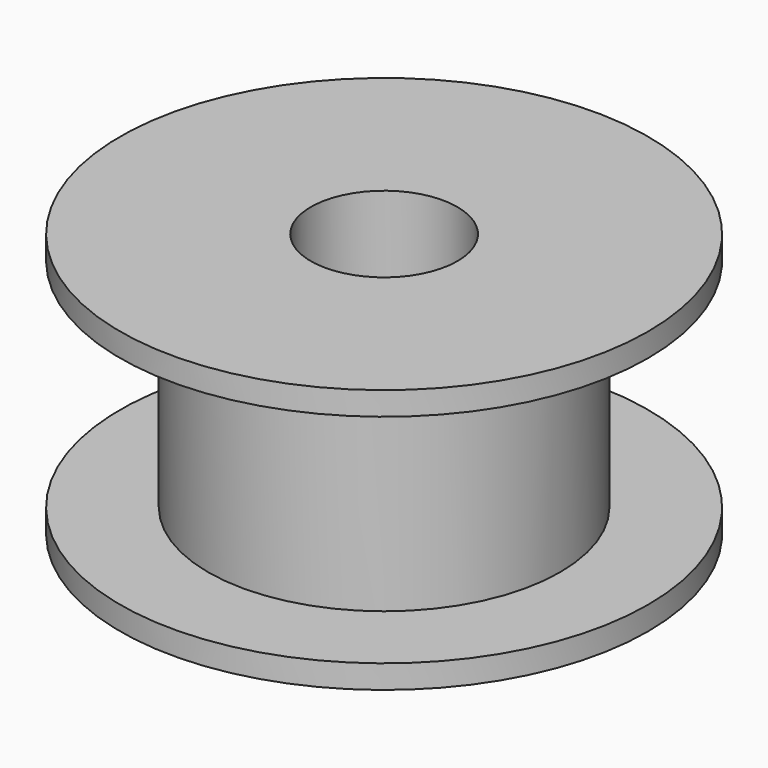
from build123d import *

# Parameters (mm, degrees)
F0_R     = 6
F1_DEPTH = 7.4
F2_R     = 9
F3_DEPTH = 0.8
F4_R     = 9
F5_DEPTH = 0.8
F6_R     = 2.5
F7_DEPTH = 9.001


# Not quite as in the source:
# - ends of sketch curves that miss each other by under 0.0002 mm in the source are joined


with BuildPart() as f1:
    # F0 (on Top) → F1 (new body)
    with BuildSketch(Plane.XY):
        Circle(F0_R)
        with BuildLine():
            ThreePointArc((0.3806045388, -5.7658808945), (0.3821052842, -5.7646171302), (0.3836035472, -5.7633504238))
            ThreePointArc((0.3836035472, -5.7633504238), (0, -5.25), (-0.3836035472, -5.7633504238))
            ThreePointArc((-0.3836035472, -5.7633504238), (-0.3821052842, -5.7646171302), (-0.3806045388, -5.7658808945))
            ThreePointArc((-0.3806045388, -5.7658808945), (-0.3463448965, -5.8591249109), (-0.4093829562, -5.9358997292))
            ThreePointArc((-0.4093829562, -5.9358997292), (-0.4525361238, -5.9421469593), (-0.4942455569, -5.9294368476))
            ThreePointArc((-0.4942455569, -5.9294368476), (-0.9311233557, -5.8766920369), (-1.3629081057, -5.7918029572))
            ThreePointArc((-1.3629081057, -5.7918029572), (-1.4044855806, -5.7906197903), (-1.441985055, -5.7726232426))
            ThreePointArc((-1.441985055, -5.7726232426), (-1.4799897199, -5.6798690996), (-1.4184467175, -5.6007480248))
            ThreePointArc((-1.4184467175, -5.6007480248), (-1.4166288992, -5.6000098693), (-1.4148125327, -5.5992681488))
            ThreePointArc((-1.4148125327, -5.5992681488), (-1.6210071809, -4.9925028678), (-2.1444698391, -5.3621881184))
            ThreePointArc((-2.1444698391, -5.3621881184), (-2.1434363401, -5.3638558164), (-2.1423995711, -5.3655214836))
            ThreePointArc((-2.1423995711, -5.3655214836), (-2.1392066719, -5.4658737363), (-2.2247634424, -5.5184171304))
            ThreePointArc((-2.2247634424, -5.5184171304), (-2.2652635999, -5.5109390447), (-2.2993151455, -5.4877727597))
            ThreePointArc((-2.2993151455, -5.4877727597), (-2.7009268548, -5.3016501323), (-3.0875904018, -5.0861857527))
            ThreePointArc((-3.0875904018, -5.0861857527), (-3.1238007071, -5.0726605298), (-3.1521764439, -5.0464129504))
            ThreePointArc((-3.1521764439, -5.0464129504), (-3.1620439351, -4.945353315), (-3.078417275, -4.8877599211))
            ThreePointArc((-3.078417275, -4.8877599211), (-3.0764603245, -4.8876196303), (-3.0745036529, -4.8874755002))
            ThreePointArc((-3.0745036529, -4.8874755002), (-3.0831056333, -4.2466897755), (-3.6951872305, -4.4365224847))
            ThreePointArc((-3.6951872305, -4.4365224847), (-3.6947196616, -4.4384279285), (-3.6942483551, -4.4403324513))
            ThreePointArc((-3.6942483551, -4.4403324513), (-3.7234373447, -4.5379012507), (-3.8230076712, -4.5592885789))
            ThreePointArc((-3.8230076712, -4.5592885789), (-3.8560268582, -4.5406730269), (-3.8797455624, -4.5111056706))
            ThreePointArc((-3.8797455624, -4.5111056706), (-4.2068112489, -4.2077593938), (-4.5102312248, -3.8807620771))
            ThreePointArc((-4.5102312248, -3.8807620771), (-4.5371123267, -3.8585413389), (-4.5547275545, -3.8284405316))
            ThreePointArc((-4.5547275545, -3.8284405316), (-4.535446501, -3.7270635192), (-4.4368176497, -3.6967088266))
            ThreePointArc((-4.4368176497, -3.6967088266), (-4.4349131269, -3.6971801331), (-4.433007683, -3.697647702))
            ThreePointArc((-4.433007683, -3.697647702), (-4.2431749738, -3.0855661048), (-4.8839606986, -3.0769641244))
            ThreePointArc((-4.8839606986, -3.0769641244), (-4.8841048286, -3.0789207959), (-4.8842451195, -3.0808777465))
            ThreePointArc((-4.8842451195, -3.0808777465), (-4.9440169669, -3.1654857116), (-5.0466911586, -3.1517310085))
            ThreePointArc((-5.0466911586, -3.1517310085), (-5.069110444, -3.1263184325), (-5.0817550004, -3.0948773992))
            ThreePointArc((-5.0817550004, -3.0948773992), (-5.3012375926, -2.7017364763), (-5.4903626511, -2.2931240611))
            ThreePointArc((-5.4903626511, -2.2931240611), (-5.5060730233, -2.2671022941), (-5.5132397924, -2.2375627347))
            ThreePointArc((-5.5132397924, -2.2375627347), (-5.4658096238, -2.1437373386), (-5.3606781484, -2.144183121))
            ThreePointArc((-5.3606781484, -2.144183121), (-5.3590124813, -2.14521989), (-5.3573447832, -2.146253389))
            ThreePointArc((-5.3573447832, -2.146253389), (-4.9876595327, -1.6227907307), (-5.5944248136, -1.4165960825))
            ThreePointArc((-5.5944248136, -1.4165960825), (-5.5951665342, -1.4184124491), (-5.5959046897, -1.4202302674))
            ThreePointArc((-5.5959046897, -1.4202302674), (-5.6812065984, -1.4824247971), (-5.7747415985, -1.4334781025))
            ThreePointArc((-5.7747415985, -1.4334781025), (-5.7857648681, -1.4063168524), (-5.7884387811, -1.3771261661))
            ThreePointArc((-5.7884387811, -1.3771261661), (-5.8767455172, -0.9307857571), (-5.9306876982, -0.4790025331))
            ThreePointArc((-5.9306876982, -0.4790025331), (-5.8853739929, -0.3594639118), (-5.7595648686, -0.3821548374))
            ThreePointArc((-5.7595648686, -0.3821548374), (-5.7583011043, -0.3836555828), (-5.7570343979, -0.3851538458))
            ThreePointArc((-5.7570343979, -0.3851538458), (-5.2436839741, -0.0015502986), (-5.7570343979, 0.3820532486))
            ThreePointArc((-5.7570343979, 0.3820532486), (-5.7583011043, 0.3805549856), (-5.7595648686, 0.3790542403))
            ThreePointArc((-5.7595648686, 0.3790542403), (-5.8622942172, 0.3468784197), (-5.9346909264, 0.426548483))
            ThreePointArc((-5.9346909264, 0.426548483), (-5.9358323151, 0.4509676612), (-5.9310148859, 0.4749341254))
            ThreePointArc((-5.9310148859, 0.4749341254), (-5.8765991635, 0.9317093277), (-5.7870583583, 1.3829156003))
            ThreePointArc((-5.7870583583, 1.3829156003), (-5.7843038364, 1.4029349854), (-5.7775807433, 1.4219918266))
            ThreePointArc((-5.7775807433, 1.4219918266), (-5.6843404021, 1.4793255219), (-5.594431999, 1.416896419))
            ThreePointArc((-5.594431999, 1.416896419), (-5.5936938435, 1.4150786007), (-5.5929521229, 1.4132622341))
            ThreePointArc((-5.5929521229, 1.4132622341), (-4.986186842, 1.6194568823), (-5.3558720925, 2.1429195405))
            ThreePointArc((-5.3558720925, 2.1429195405), (-5.3575397905, 2.1418860415), (-5.3592054577, 2.1408492726))
            ThreePointArc((-5.3592054577, 2.1408492726), (-5.4688284086, 2.1433207754), (-5.5102834557, 2.2448332315))
            ThreePointArc((-5.5102834557, 2.2448332315), (-5.5046167329, 2.2637285902), (-5.4953509969, 2.2811438842))
            ThreePointArc((-5.4953509969, 2.2811438842), (-5.3005253653, 2.7031335247), (-5.0733549953, 3.1086281688))
            ThreePointArc((-5.0733549953, 3.1086281688), (-5.0663266491, 3.1222793914), (-5.0572912917, 3.1346937317))
            ThreePointArc((-5.0572912917, 3.1346937317), (-4.9499559959, 3.164809758), (-4.8814438952, 3.0768669764))
            ThreePointArc((-4.8814438952, 3.0768669764), (-4.8813036044, 3.0749100259), (-4.8811594743, 3.0729533544))
            ThreePointArc((-4.8811594743, 3.0729533544), (-4.2403737496, 3.0815553348), (-4.4302064588, 3.6936369319))
            ThreePointArc((-4.4302064588, 3.6936369319), (-4.4321119026, 3.693169363), (-4.4340164255, 3.6926980566))
            ThreePointArc((-4.4340164255, 3.6926980566), (-4.538656044, 3.7304491107), (-4.5436525599, 3.841577985))
            ThreePointArc((-4.5436525599, 3.841577985), (-4.5343248359, 3.8545144167), (-4.523059132, 3.8658034209))
            ThreePointArc((-4.523059132, 3.8658034209), (-4.2049856642, 4.2095837756), (-3.8608578947, 4.5272813384))
            ThreePointArc((-3.8608578947, 4.5272813384), (-3.852175731, 4.5356041669), (-3.8425571832, 4.5428244841))
            ThreePointArc((-3.8425571832, 4.5428244841), (-3.729720065, 4.5410442426), (-3.6903928007, 4.4352673511))
            ThreePointArc((-3.6903928007, 4.4352673511), (-3.6908641072, 4.4333628283), (-3.6913316761, 4.4314573845))
            ThreePointArc((-3.6913316761, 4.4314573845), (-3.0792500789, 4.2416246753), (-3.0706480985, 4.8824104))
            ThreePointArc((-3.0706480985, 4.8824104), (-3.0726047701, 4.8825545301), (-3.0745617206, 4.8826948209))
            ThreePointArc((-3.0745617206, 4.8826948209), (-3.1626644803, 4.9516976688), (-3.1315994665, 5.0592079204))
            ThreePointArc((-3.1315994665, 5.0592079204), (-3.119936027, 5.0676010486), (-3.1071900735, 5.074235888))
            ThreePointArc((-3.1071900735, 5.074235888), (-2.6977366196, 5.3032741897), (-2.2715103211, 5.4993400387))
            ThreePointArc((-2.2715103211, 5.4993400387), (-2.1503267928, 5.4810489954), (-2.1378670951, 5.3591278498))
            ThreePointArc((-2.1378670951, 5.3591278498), (-2.1389038641, 5.3574621827), (-2.1399373631, 5.3557944847))
            ThreePointArc((-2.1399373631, 5.3557944847), (-1.6164747048, 4.9861092341), (-1.4102800566, 5.592874515))
            ThreePointArc((-1.4102800566, 5.592874515), (-1.4120964232, 5.5936162356), (-1.4139142415, 5.5943543911))
            ThreePointArc((-1.4139142415, 5.5943543911), (-1.4763804938, 5.6864908439), (-1.4149370546, 5.7793125137))
            ThreePointArc((-1.4149370546, 5.7793125137), (-1.3999049739, 5.7842378178), (-1.3842842971, 5.7867311139))
            ThreePointArc((-1.3842842971, 5.7867311139), (-0.9264014664, 5.8774382449), (-0.4628171036, 5.9319727181))
            ThreePointArc((-0.4628171036, 5.9319727181), (-0.4476995944, 5.9342860016), (-0.4324061315, 5.9342670093))
            ThreePointArc((-0.4324061315, 5.9342670093), (-0.3449604214, 5.8651285474), (-0.3758388115, 5.7580145701))
            ThreePointArc((-0.3758388115, 5.7580145701), (-0.3773395569, 5.7567508057), (-0.3788378199, 5.7554840994))
            ThreePointArc((-0.3788378199, 5.7554840994), (0.0047657273, 5.2421336756), (0.3883692745, 5.7554840994))
            ThreePointArc((0.3883692745, 5.7554840994), (0.3868710115, 5.7567508057), (0.3853702662, 5.7580145701))
            ThreePointArc((0.3853702662, 5.7580145701), (0.3538873578, 5.8631766757), (0.4378708106, 5.9338662905))
            ThreePointArc((0.4378708106, 5.9338662905), (0.4573929959, 5.9342736516), (0.4766221718, 5.9308794715))
            ThreePointArc((0.4766221718, 5.9308794715), (0.9358457669, 5.8759418565), (1.3894149145, 5.785501378))
            ThreePointArc((1.3894149145, 5.785501378), (1.4093589983, 5.7827272829), (1.4283429976, 5.7760138748))
            ThreePointArc((1.4283429976, 5.7760138748), (1.4856410056, 5.6827706834), (1.4232124448, 5.5928817004))
            ThreePointArc((1.4232124448, 5.5928817004), (1.4213946265, 5.5921435449), (1.41957826, 5.5914018243))
            ThreePointArc((1.41957826, 5.5914018243), (1.6257729082, 4.9846365434), (2.1492355664, 5.3543217939))
            ThreePointArc((2.1492355664, 5.3543217939), (2.1482020674, 5.355989492), (2.1471652984, 5.3576551591))
            ThreePointArc((2.1471652984, 5.3576551591), (2.1484055829, 5.4654463163), (2.2467992931, 5.5094820933))
            ThreePointArc((2.2467992931, 5.5094820933), (2.2701462131, 5.5030245881), (2.2912554418, 5.4911427318))
            ThreePointArc((2.2912554418, 5.4911427318), (2.7064393495, 5.298838179), (3.1056182667, 5.0751980436))
            ThreePointArc((3.1056182667, 5.0751980436), (3.1286854235, 5.0647208158), (3.1483792489, 5.048782834))
            ThreePointArc((3.1483792489, 5.048782834), (3.169420639, 4.9436317748), (3.0831830023, 4.8798935967))
            ThreePointArc((3.0831830023, 4.8798935967), (3.0812260518, 4.8797533058), (3.0792693802, 4.8796091758))
            ThreePointArc((3.0792693802, 4.8796091758), (3.0878713606, 4.238823451), (3.6999529578, 4.4286561602))
            ThreePointArc((3.6999529578, 4.4286561602), (3.6994853889, 4.4305616041), (3.6990140824, 4.4324661269))
            ThreePointArc((3.6990140824, 4.4324661269), (3.7316088821, 4.5330409603), (3.8362478957, 4.5481537004))
            ThreePointArc((3.8362478957, 4.5481537004), (3.8609061096, 4.53271015), (3.8800750956, 4.5108222369))
            ThreePointArc((3.8800750956, 4.5108222369), (4.2117676312, 4.2027982846), (4.5190837616, 3.8704498389))
            ThreePointArc((4.5190837616, 3.8704498389), (4.5419784366, 3.8505567927), (4.5578563234, 3.8247151182))
            ThreePointArc((4.5578563234, 3.8247151182), (4.5416785998, 3.7208726241), (4.441583377, 3.6888425022))
            ThreePointArc((4.441583377, 3.6888425022), (4.4396788542, 3.6893138086), (4.4377734103, 3.6897813775))
            ThreePointArc((4.4377734103, 3.6897813775), (4.2479407012, 3.0776997804), (4.8887264259, 3.0690978))
            ThreePointArc((4.8887264259, 3.0690978), (4.8888705559, 3.0710544715), (4.8890108468, 3.073011422))
            ThreePointArc((4.8890108468, 3.073011422), (4.9489466875, 3.1576907408), (5.0517351443, 3.1436399335))
            ThreePointArc((5.0517351443, 3.1436399335), (5.0739585149, 3.1183183587), (5.0865115484, 3.0870536549))
            ThreePointArc((5.0865115484, 3.0870536549), (5.3044458004, 2.6954322011), (5.4922842876, 2.2885177089))
            ThreePointArc((5.4922842876, 2.2885177089), (5.5108977286, 2.2590924146), (5.5182939971, 2.2250688442))
            ThreePointArc((5.5182939971, 2.2250688442), (5.4685840303, 2.1346836809), (5.3654438757, 2.1363167965))
            ThreePointArc((5.3654438757, 2.1363167965), (5.3637782086, 2.1373535655), (5.3621105105, 2.1383870645))
            ThreePointArc((5.3621105105, 2.1383870645), (4.99242526, 1.6149244063), (5.5991905409, 1.4087297581))
            ThreePointArc((5.5991905409, 1.4087297581), (5.5999322615, 1.4105461246), (5.600670417, 1.4123639429))
            ThreePointArc((5.600670417, 1.4123639429), (5.6817933965, 1.4741605567), (5.7749452179, 1.4326575759))
            ThreePointArc((5.7749452179, 1.4326575759), (5.7905658496, 1.3983050131), (5.7923433498, 1.3606096128))
            ThreePointArc((5.7923433498, 1.3606096128), (5.8777300273, 0.9245483905), (5.9303365162, 0.4833309479))
            ThreePointArc((5.9303365162, 0.4833309479), (5.9406046173, 0.4461148884), (5.9360098784, 0.407782691))
            ThreePointArc((5.9360098784, 0.407782691), (5.8600341125, 0.3404768743), (5.7643305959, 0.374288513))
            ThreePointArc((5.7643305959, 0.374288513), (5.7630668316, 0.3757892583), (5.7618001253, 0.3772875213))
            ThreePointArc((5.7618001253, 0.3772875213), (5.2484497014, -0.0063160259), (5.7618001253, -0.3899195731))
            ThreePointArc((5.7618001253, -0.3899195731), (5.7630668316, -0.3884213101), (5.7643305959, -0.3869205647))
            ThreePointArc((5.7643305959, -0.3869205647), (5.8589130817, -0.352896847), (5.9352813712, -0.4182523696))
            ThreePointArc((5.9352813712, -0.4182523696), (5.9405882849, -0.4589613406), (5.9290914374, -0.4983720771))
            ThreePointArc((5.9290914374, -0.4983720771), (5.8758462536, -0.9364458362), (5.7902789498, -1.3693683519))
            ThreePointArc((5.7902789498, -1.3693683519), (5.7890432658, -1.4109094735), (5.7710268611, -1.4483607867))
            ThreePointArc((5.7710268611, -1.4483607867), (5.6782814399, -1.4863006219), (5.5991977263, -1.4247627434))
            ThreePointArc((5.5991977263, -1.4247627434), (5.5984595708, -1.4229449251), (5.5977178502, -1.4211285585))
            ThreePointArc((5.5977178502, -1.4211285585), (4.9909525693, -1.6273232067), (5.3606378198, -2.150785865))
            ThreePointArc((5.3606378198, -2.150785865), (5.3623055179, -2.149752366), (5.363971185, -2.148715597))
            ThreePointArc((5.363971185, -2.148715597), (5.4965423161, -2.1730904294), (5.4844051341, -2.3073361968))
            ThreePointArc((5.4844051341, -2.3073361968), (5.2993121671, -2.705511145), (5.0853590441, -3.0889518275))
            ThreePointArc((5.0853590441, -3.0889518275), (5.0710792206, -3.130167057), (5.0406318988, -3.1614126685))
            ThreePointArc((5.0406318988, -3.1614126685), (4.9414861677, -3.167246403), (4.8862096226, -3.0847333009))
            ThreePointArc((4.8862096226, -3.0847333009), (4.8860693317, -3.0827763503), (4.8859252016, -3.0808196788))
            ThreePointArc((4.8859252016, -3.0808196788), (4.2451394769, -3.0894216592), (4.4349721861, -3.7015032564))
            ThreePointArc((4.4349721861, -3.7015032564), (4.43687763, -3.7010356874), (4.4387821528, -3.700564381))
            ThreePointArc((4.4387821528, -3.700564381), (4.5338661391, -3.7271588755), (4.5597701404, -3.8224332913))
            ThreePointArc((4.5597701404, -3.8224332913), (4.2049311669, -4.2096382127), (3.8173294995, -4.5640437653))
            ThreePointArc((3.8173294995, -4.5640437653), (3.7218637964, -4.5383274637), (3.695158528, -4.4431336756))
            ThreePointArc((3.695158528, -4.4431336756), (3.6956298345, -4.4412291528), (3.6960974034, -4.4393237089))
            ThreePointArc((3.6960974034, -4.4393237089), (3.0840158062, -4.2494909997), (3.0754138259, -4.8902767244))
            ThreePointArc((3.0754138259, -4.8902767244), (3.0773704974, -4.8904208545), (3.0793274479, -4.8905611454))
            ThreePointArc((3.0793274479, -4.8905611454), (3.1614118111, -4.944984516), (3.1570355374, -5.0433745266))
            ThreePointArc((3.1570355374, -5.0433745266), (2.6997840023, -5.3022322036), (2.2214782118, -5.5197404427))
            ThreePointArc((2.2214782118, -5.5197404427), (2.1386184867, -5.4657888682), (2.1426328224, -5.3669941743))
            ThreePointArc((2.1426328224, -5.3669941743), (2.1436695914, -5.3653285072), (2.1447030904, -5.3636608091))
            ThreePointArc((2.1447030904, -5.3636608091), (1.6212404321, -4.9939755586), (1.4150457839, -5.6007408395))
            ThreePointArc((1.4150457839, -5.6007408395), (1.4168621505, -5.6014825601), (1.4186799688, -5.6022207156))
            ThreePointArc((1.4186799688, -5.6022207156), (1.4799653708, -5.6795779085), (1.4450020565, -5.7718687664))
            ThreePointArc((1.4450020565, -5.7718687664), (0.9728192286, -5.8699337942), (0.4942455569, -5.9294368476))
            ThreePointArc((0.4942455569, -5.9294368476), (0.4525361238, -5.9421469593), (0.4093829562, -5.9358997292))
            ThreePointArc((0.4093829562, -5.9358997292), (0.3463448965, -5.8591249109), (0.3806045388, -5.7658808945))
        make_face(mode=Mode.SUBTRACT)
        with BuildLine():
            ThreePointArc((-0.3836035472, -5.7633504238), (0, -5.25), (0.3836035472, -5.7633504238))
            ThreePointArc((0.3836035472, -5.7633504238), (0.3821052842, -5.7646171302), (0.3806045388, -5.7658808945))
            ThreePointArc((0.3806045388, -5.7658808945), (0.3463448965, -5.8591249109), (0.4093829562, -5.9358997292))
            ThreePointArc((0.4093829562, -5.9358997292), (0.4518258123, -5.9328200238), (0.4942455569, -5.9294368476))
            ThreePointArc((0.4942455569, -5.9294368476), (0.9728192286, -5.8699337942), (1.4450020565, -5.7718687664))
            ThreePointArc((1.4450020565, -5.7718687664), (1.4799653708, -5.6795779085), (1.4186799688, -5.6022207156))
            ThreePointArc((1.4186799688, -5.6022207156), (1.4168621505, -5.6014825601), (1.4150457839, -5.6007408395))
            ThreePointArc((1.4150457839, -5.6007408395), (1.6212404321, -4.9939755586), (2.1447030904, -5.3636608091))
            ThreePointArc((2.1447030904, -5.3636608091), (2.1436695914, -5.3653285072), (2.1426328224, -5.3669941743))
            ThreePointArc((2.1426328224, -5.3669941743), (2.1386184867, -5.4657888682), (2.2214782118, -5.5197404427))
            ThreePointArc((2.2214782118, -5.5197404427), (2.6997840023, -5.3022322036), (3.1570355374, -5.0433745266))
            ThreePointArc((3.1570355374, -5.0433745266), (3.1614118111, -4.944984516), (3.0793274479, -4.8905611454))
            ThreePointArc((3.0793274479, -4.8905611454), (3.0773704974, -4.8904208545), (3.0754138259, -4.8902767244))
            ThreePointArc((3.0754138259, -4.8902767244), (3.0840158062, -4.2494909997), (3.6960974034, -4.4393237089))
            ThreePointArc((3.6960974034, -4.4393237089), (3.6956298345, -4.4412291528), (3.695158528, -4.4431336756))
            ThreePointArc((3.695158528, -4.4431336756), (3.7218637964, -4.5383274637), (3.8173294995, -4.5640437653))
            ThreePointArc((3.8173294995, -4.5640437653), (4.2049311669, -4.2096382127), (4.5597701404, -3.8224332913))
            ThreePointArc((4.5597701404, -3.8224332913), (4.5338661391, -3.7271588755), (4.4387821528, -3.700564381))
            ThreePointArc((4.4387821528, -3.700564381), (4.43687763, -3.7010356874), (4.4349721861, -3.7015032564))
            ThreePointArc((4.4349721861, -3.7015032564), (4.2451394769, -3.0894216592), (4.8859252016, -3.0808196788))
            ThreePointArc((4.8859252016, -3.0808196788), (4.8860693317, -3.0827763503), (4.8862096226, -3.0847333009))
            ThreePointArc((4.8862096226, -3.0847333009), (4.9414861677, -3.167246403), (5.0406318988, -3.1614126685))
            ThreePointArc((5.0406318988, -3.1614126685), (5.0631251009, -3.125262263), (5.0853590441, -3.0889518275))
            ThreePointArc((5.0853590441, -3.0889518275), (5.2993121671, -2.705511145), (5.4844051341, -2.3073361968))
            ThreePointArc((5.4844051341, -2.3073361968), (5.4965423161, -2.1730904294), (5.363971185, -2.148715597))
            ThreePointArc((5.363971185, -2.148715597), (5.3623055179, -2.149752366), (5.3606378198, -2.150785865))
            ThreePointArc((5.3606378198, -2.150785865), (4.9909525693, -1.6273232067), (5.5977178502, -1.4211285585))
            ThreePointArc((5.5977178502, -1.4211285585), (5.5984595708, -1.4229449251), (5.5991977263, -1.4247627434))
            ThreePointArc((5.5991977263, -1.4247627434), (5.6782814399, -1.4863006219), (5.7710268611, -1.4483607867))
            ThreePointArc((5.7710268611, -1.4483607867), (5.7807878325, -1.4088974538), (5.7902789498, -1.3693683519))
            ThreePointArc((5.7902789498, -1.3693683519), (5.8758462536, -0.9364458362), (5.9290914374, -0.4983720771))
            ThreePointArc((5.9290914374, -0.4983720771), (5.9323216642, -0.4583226733), (5.9352813712, -0.4182523696))
            ThreePointArc((5.9352813712, -0.4182523696), (5.8589130817, -0.352896847), (5.7643305959, -0.3869205647))
            ThreePointArc((5.7643305959, -0.3869205647), (5.7630668316, -0.3884213101), (5.7618001253, -0.3899195731))
            ThreePointArc((5.7618001253, -0.3899195731), (5.2484497014, -0.0063160259), (5.7618001253, 0.3772875213))
            ThreePointArc((5.7618001253, 0.3772875213), (5.7630668316, 0.3757892583), (5.7643305959, 0.374288513))
            ThreePointArc((5.7643305959, 0.374288513), (5.8600341125, 0.3404768743), (5.9360098784, 0.407782691))
            ThreePointArc((5.9360098784, 0.407782691), (5.9332934424, 0.4455658494), (5.9303365162, 0.4833309479))
            ThreePointArc((5.9303365162, 0.4833309479), (5.8777300273, 0.9245483905), (5.7923433498, 1.3606096128))
            ThreePointArc((5.7923433498, 1.3606096128), (5.7837564722, 1.3966606856), (5.7749452179, 1.4326575759))
            ThreePointArc((5.7749452179, 1.4326575759), (5.6817933965, 1.4741605567), (5.600670417, 1.4123639429))
            ThreePointArc((5.600670417, 1.4123639429), (5.5999322615, 1.4105461246), (5.5991905409, 1.4087297581))
            ThreePointArc((5.5991905409, 1.4087297581), (4.99242526, 1.6149244063), (5.3621105105, 2.1383870645))
            ThreePointArc((5.3621105105, 2.1383870645), (5.3637782086, 2.1373535655), (5.3654438757, 2.1363167965))
            ThreePointArc((5.3654438757, 2.1363167965), (5.4685840303, 2.1346836809), (5.5182939971, 2.2250688442))
            ThreePointArc((5.5182939971, 2.2250688442), (5.5053805482, 2.2568307467), (5.4922842876, 2.2885177089))
            ThreePointArc((5.4922842876, 2.2885177089), (5.3044458004, 2.6954322011), (5.0865115484, 3.0870536549))
            ThreePointArc((5.0865115484, 3.0870536549), (5.0692023043, 3.1153953197), (5.0517351443, 3.1436399335))
            ThreePointArc((5.0517351443, 3.1436399335), (4.9489466875, 3.1576907408), (4.8890108468, 3.073011422))
            ThreePointArc((4.8890108468, 3.073011422), (4.8888705559, 3.0710544715), (4.8887264259, 3.0690978))
            ThreePointArc((4.8887264259, 3.0690978), (4.2479407012, 3.0776997804), (4.4377734103, 3.6897813775))
            ThreePointArc((4.4377734103, 3.6897813775), (4.4396788542, 3.6893138086), (4.441583377, 3.6888425022))
            ThreePointArc((4.441583377, 3.6888425022), (4.5416785998, 3.7208726241), (4.5578563234, 3.8247151182))
            ThreePointArc((4.5578563234, 3.8247151182), (4.5385276514, 3.8476313177), (4.5190837616, 3.8704498389))
            ThreePointArc((4.5190837616, 3.8704498389), (4.2117676312, 4.2027982846), (3.8800750956, 4.5108222369))
            ThreePointArc((3.8800750956, 4.5108222369), (3.8582066477, 4.5295409772), (3.8362478957, 4.5481537004))
            ThreePointArc((3.8362478957, 4.5481537004), (3.7316088821, 4.5330409603), (3.6990140824, 4.4324661269))
            ThreePointArc((3.6990140824, 4.4324661269), (3.6994853889, 4.4305616041), (3.6999529578, 4.4286561602))
            ThreePointArc((3.6999529578, 4.4286561602), (3.0878713606, 4.238823451), (3.0792693802, 4.8796091758))
            ThreePointArc((3.0792693802, 4.8796091758), (3.0812260518, 4.8797533058), (3.0831830023, 4.8798935967))
            ThreePointArc((3.0831830023, 4.8798935967), (3.169420639, 4.9436317748), (3.1483792489, 5.048782834))
            ThreePointArc((3.1483792489, 5.048782834), (3.1270266504, 5.0620355913), (3.1056182667, 5.0751980436))
            ThreePointArc((3.1056182667, 5.0751980436), (2.7064393495, 5.298838179), (2.2912554418, 5.4911427318))
            ThreePointArc((2.2912554418, 5.4911427318), (2.2690458958, 5.5003573268), (2.2467992931, 5.5094820933))
            ThreePointArc((2.2467992931, 5.5094820933), (2.1484055829, 5.4654463163), (2.1471652984, 5.3576551591))
            ThreePointArc((2.1471652984, 5.3576551591), (2.1482020674, 5.355989492), (2.1492355664, 5.3543217939))
            ThreePointArc((2.1492355664, 5.3543217939), (1.6257729082, 4.9846365434), (1.41957826, 5.5914018243))
            ThreePointArc((1.41957826, 5.5914018243), (1.4213946265, 5.5921435449), (1.4232124448, 5.5928817004))
            ThreePointArc((1.4232124448, 5.5928817004), (1.4856410056, 5.6827706834), (1.4283429976, 5.7760138748))
            ThreePointArc((1.4283429976, 5.7760138748), (1.4088869422, 5.7807903944), (1.3894149145, 5.785501378))
            ThreePointArc((1.3894149145, 5.785501378), (0.9358457669, 5.8759418565), (0.4766221718, 5.9308794715))
            ThreePointArc((0.4766221718, 5.9308794715), (0.45724893, 5.9324045223), (0.4378708106, 5.9338662905))
            ThreePointArc((0.4378708106, 5.9338662905), (0.3538873578, 5.8631766757), (0.3853702662, 5.7580145701))
            ThreePointArc((0.3853702662, 5.7580145701), (0.3868710115, 5.7567508057), (0.3883692745, 5.7554840994))
            ThreePointArc((0.3883692745, 5.7554840994), (0.0047657273, 5.2421336756), (-0.3788378199, 5.7554840994))
            ThreePointArc((-0.3788378199, 5.7554840994), (-0.3773395569, 5.7567508057), (-0.3758388115, 5.7580145701))
            ThreePointArc((-0.3758388115, 5.7580145701), (-0.3449604214, 5.8651285474), (-0.4324061315, 5.9342670093))
            ThreePointArc((-0.4324061315, 5.9342670093), (-0.4476130875, 5.9331393481), (-0.4628171036, 5.9319727181))
            ThreePointArc((-0.4628171036, 5.9319727181), (-0.9264014664, 5.8774382449), (-1.3842842971, 5.7867311139))
            ThreePointArc((-1.3842842971, 5.7867311139), (-1.3996155911, 5.7830421231), (-1.4149370546, 5.7793125137))
            ThreePointArc((-1.4149370546, 5.7793125137), (-1.4763804938, 5.6864908439), (-1.4139142415, 5.5943543911))
            ThreePointArc((-1.4139142415, 5.5943543911), (-1.4120964232, 5.5936162356), (-1.4102800566, 5.592874515))
            ThreePointArc((-1.4102800566, 5.592874515), (-1.6164747048, 4.9861092341), (-2.1399373631, 5.3557944847))
            ThreePointArc((-2.1399373631, 5.3557944847), (-2.1389038641, 5.3574621827), (-2.1378670951, 5.3591278498))
            ThreePointArc((-2.1378670951, 5.3591278498), (-2.1503267928, 5.4810489954), (-2.2715103211, 5.4993400387))
            ThreePointArc((-2.2715103211, 5.4993400387), (-2.6977366196, 5.3032741897), (-3.1071900735, 5.074235888))
            ThreePointArc((-3.1071900735, 5.074235888), (-3.1194038198, 5.0667366035), (-3.1315994665, 5.0592079204))
            ThreePointArc((-3.1315994665, 5.0592079204), (-3.1626644803, 4.9516976688), (-3.0745617206, 4.8826948209))
            ThreePointArc((-3.0745617206, 4.8826948209), (-3.0726047701, 4.8825545301), (-3.0706480985, 4.8824104))
            ThreePointArc((-3.0706480985, 4.8824104), (-3.0792500789, 4.2416246753), (-3.6913316761, 4.4314573845))
            ThreePointArc((-3.6913316761, 4.4314573845), (-3.6908641072, 4.4333628283), (-3.6903928007, 4.4352673511))
            ThreePointArc((-3.6903928007, 4.4352673511), (-3.729720065, 4.5410442426), (-3.8425571832, 4.5428244841))
            ThreePointArc((-3.8425571832, 4.5428244841), (-3.8517153793, 4.5350621426), (-3.8608578947, 4.5272813384))
            ThreePointArc((-3.8608578947, 4.5272813384), (-4.2049856642, 4.2095837756), (-4.523059132, 3.8658034209))
            ThreePointArc((-4.523059132, 3.8658034209), (-4.533372028, 3.8537044588), (-4.5436525599, 3.841577985))
            ThreePointArc((-4.5436525599, 3.841577985), (-4.538656044, 3.7304491107), (-4.4340164255, 3.6926980566))
            ThreePointArc((-4.4340164255, 3.6926980566), (-4.4321119026, 3.693169363), (-4.4302064588, 3.6936369319))
            ThreePointArc((-4.4302064588, 3.6936369319), (-4.2403737496, 3.0815553348), (-4.8811594743, 3.0729533544))
            ThreePointArc((-4.8811594743, 3.0729533544), (-4.8813036044, 3.0749100259), (-4.8814438952, 3.0768669764))
            ThreePointArc((-4.8814438952, 3.0768669764), (-4.9499559959, 3.164809758), (-5.0572912917, 3.1346937317))
            ThreePointArc((-5.0572912917, 3.1346937317), (-5.0653399097, 3.121671283), (-5.0733549953, 3.1086281688))
            ThreePointArc((-5.0733549953, 3.1086281688), (-5.3005253653, 2.7031335247), (-5.4953509969, 2.2811438842))
            ThreePointArc((-5.4953509969, 2.2811438842), (-5.502847176, 2.2630008744), (-5.5102834557, 2.2448332315))
            ThreePointArc((-5.5102834557, 2.2448332315), (-5.4688284086, 2.1433207754), (-5.3592054577, 2.1408492726))
            ThreePointArc((-5.3592054577, 2.1408492726), (-5.3575397905, 2.1418860415), (-5.3558720925, 2.1429195405))
            ThreePointArc((-5.3558720925, 2.1429195405), (-4.986186842, 1.6194568823), (-5.5929521229, 1.4132622341))
            ThreePointArc((-5.5929521229, 1.4132622341), (-5.5936938435, 1.4150786007), (-5.594431999, 1.416896419))
            ThreePointArc((-5.594431999, 1.416896419), (-5.6843404021, 1.4793255219), (-5.7775807433, 1.4219918266))
            ThreePointArc((-5.7775807433, 1.4219918266), (-5.7823525598, 1.4024617195), (-5.7870583583, 1.3829156003))
            ThreePointArc((-5.7870583583, 1.3829156003), (-5.8765991635, 0.9317093277), (-5.9310148859, 0.4749341254))
            ThreePointArc((-5.9310148859, 0.4749341254), (-5.9329022323, 0.4507450517), (-5.9346909264, 0.426548483))
            ThreePointArc((-5.9346909264, 0.426548483), (-5.8622942172, 0.3468784197), (-5.7595648686, 0.3790542403))
            ThreePointArc((-5.7595648686, 0.3790542403), (-5.7583011043, 0.3805549856), (-5.7570343979, 0.3820532486))
            ThreePointArc((-5.7570343979, 0.3820532486), (-5.2436839741, -0.0015502986), (-5.7570343979, -0.3851538458))
            ThreePointArc((-5.7570343979, -0.3851538458), (-5.7583011043, -0.3836555828), (-5.7595648686, -0.3821548374))
            ThreePointArc((-5.7595648686, -0.3821548374), (-5.8853739929, -0.3594639118), (-5.9306876982, -0.4790025331))
            ThreePointArc((-5.9306876982, -0.4790025331), (-5.8767455172, -0.9307857571), (-5.7884387811, -1.3771261661))
            ThreePointArc((-5.7884387811, -1.3771261661), (-5.7816588457, -1.4053188221), (-5.7747415985, -1.4334781025))
            ThreePointArc((-5.7747415985, -1.4334781025), (-5.6812065984, -1.4824247971), (-5.5959046897, -1.4202302674))
            ThreePointArc((-5.5959046897, -1.4202302674), (-5.5951665342, -1.4184124491), (-5.5944248136, -1.4165960825))
            ThreePointArc((-5.5944248136, -1.4165960825), (-4.9876595327, -1.6227907307), (-5.3573447832, -2.146253389))
            ThreePointArc((-5.3573447832, -2.146253389), (-5.3590124813, -2.14521989), (-5.3606781484, -2.144183121))
            ThreePointArc((-5.3606781484, -2.144183121), (-5.4658096238, -2.1437373386), (-5.5132397924, -2.2375627347))
            ThreePointArc((-5.5132397924, -2.2375627347), (-5.5018713588, -2.2653722765), (-5.4903626511, -2.2931240611))
            ThreePointArc((-5.4903626511, -2.2931240611), (-5.3012375926, -2.7017364763), (-5.0817550004, -3.0948773992))
            ThreePointArc((-5.0817550004, -3.0948773992), (-5.0643028624, -3.1233534091), (-5.0466911586, -3.1517310085))
            ThreePointArc((-5.0466911586, -3.1517310085), (-4.9440169669, -3.1654857116), (-4.8842451195, -3.0808777465))
            ThreePointArc((-4.8842451195, -3.0808777465), (-4.8841048286, -3.0789207959), (-4.8839606986, -3.0769641244))
            ThreePointArc((-4.8839606986, -3.0769641244), (-4.2431749738, -3.0855661048), (-4.433007683, -3.697647702))
            ThreePointArc((-4.433007683, -3.697647702), (-4.4349131269, -3.6971801331), (-4.4368176497, -3.6967088266))
            ThreePointArc((-4.4368176497, -3.6967088266), (-4.535446501, -3.7270635192), (-4.5547275545, -3.8284405316))
            ThreePointArc((-4.5547275545, -3.8284405316), (-4.532554887, -3.8546655103), (-4.5102312248, -3.8807620771))
            ThreePointArc((-4.5102312248, -3.8807620771), (-4.2068112489, -4.2077593938), (-3.8797455624, -4.5111056706))
            ThreePointArc((-3.8797455624, -4.5111056706), (-3.8514519655, -4.5352858518), (-3.8230076712, -4.5592885789))
            ThreePointArc((-3.8230076712, -4.5592885789), (-3.7234373447, -4.5379012507), (-3.6942483551, -4.4403324513))
            ThreePointArc((-3.6942483551, -4.4403324513), (-3.6947196616, -4.4384279285), (-3.6951872305, -4.4365224847))
            ThreePointArc((-3.6951872305, -4.4365224847), (-3.0831056333, -4.2466897755), (-3.0745036529, -4.8874755002))
            ThreePointArc((-3.0745036529, -4.8874755002), (-3.0764603245, -4.8876196303), (-3.078417275, -4.8877599211))
            ThreePointArc((-3.078417275, -4.8877599211), (-3.1620439351, -4.945353315), (-3.1521764439, -5.0464129504))
            ThreePointArc((-3.1521764439, -5.0464129504), (-3.119946801, -5.0664022697), (-3.0875904018, -5.0861857527))
            ThreePointArc((-3.0875904018, -5.0861857527), (-2.7009268548, -5.3016501323), (-2.2993151455, -5.4877727597))
            ThreePointArc((-2.2993151455, -5.4877727597), (-2.2620911867, -5.5032211897), (-2.2247634424, -5.5184171304))
            ThreePointArc((-2.2247634424, -5.5184171304), (-2.1392066719, -5.4658737363), (-2.1423995711, -5.3655214836))
            ThreePointArc((-2.1423995711, -5.3655214836), (-2.1434363401, -5.3638558164), (-2.1444698391, -5.3621881184))
            ThreePointArc((-2.1444698391, -5.3621881184), (-1.6210071809, -4.9925028678), (-1.4148125327, -5.5992681488))
            ThreePointArc((-1.4148125327, -5.5992681488), (-1.4166288992, -5.6000098693), (-1.4184467175, -5.6007480248))
            ThreePointArc((-1.4184467175, -5.6007480248), (-1.4799897199, -5.6798690996), (-1.441985055, -5.7726232426))
            ThreePointArc((-1.441985055, -5.7726232426), (-1.4024793674, -5.7823482794), (-1.3629081057, -5.7918029572))
            ThreePointArc((-1.3629081057, -5.7918029572), (-0.9311233557, -5.8766920369), (-0.4942455569, -5.9294368476))
            ThreePointArc((-0.4942455569, -5.9294368476), (-0.4518258123, -5.9328200238), (-0.4093829562, -5.9358997292))
            ThreePointArc((-0.4093829562, -5.9358997292), (-0.3463448965, -5.8591249109), (-0.3806045388, -5.7658808945))
            ThreePointArc((-0.3806045388, -5.7658808945), (-0.3821052842, -5.7646171302), (-0.3836035472, -5.7633504238))
        make_face()
    extrude(amount=F1_DEPTH)

    # F2 (on face) → F3 (join)
    with BuildSketch(Plane.XY.offset(7.4)):
        Circle(F2_R)
    extrude(amount=F3_DEPTH)

    # F4 (on face) → F5 (join)
    with BuildSketch(Plane(origin=(0, 0, 0), x_dir=(1, 0, 0), z_dir=(0, 0, -1))):
        Circle(F4_R)
    extrude(amount=F5_DEPTH)

    # F6 (on face) → F7 (cut, through all)
    with BuildSketch(Plane(origin=(0, 0, -0.8), x_dir=(1, 0, 0), z_dir=(0, 0, -1))):
        Circle(F6_R)
    extrude(amount=-F7_DEPTH, mode=Mode.SUBTRACT)


solid = f1.part
